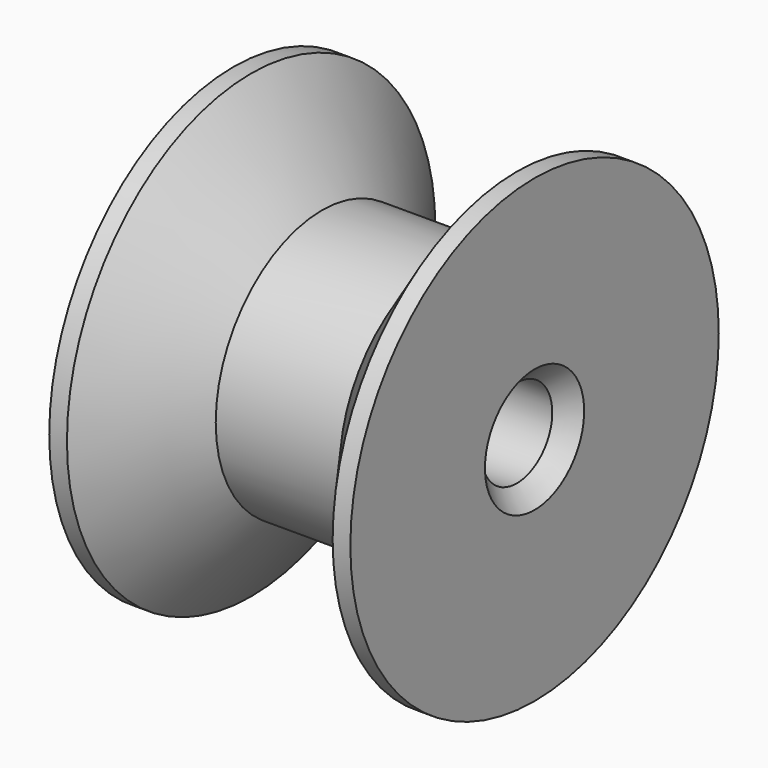
from build123d import *

# Parameters (mm, degrees)
F2_SIZE2 = 10.99999
F2_SIZE  = 7.99999
F3_SIZE  = 2


# Not quite as in the source:
# - a fillet or chamfer is up to 0.001 mm smaller than in the source, because OpenCascade refuses the exact size


with BuildPart() as f1:
    # F0 (on Front) → F1 (revolve)
    with BuildSketch(Plane.XZ):
        Polygon((0, 26), (0, 5), (34, 5), (34, 26), (32, 26), (32, 15), (2, 15), (2, 26), align=None)
    revolve(axis=Axis((17, 0, 0), (1, 0, 0)))

    # F2 (size 8 and 11 in the source; OpenCascade refuses exactly that, so slightly less here)
    f2_edges = [f1.edges().sort_by_distance(p)[0] for p in [
        (2, 0, -15),
        (32, 0, -15),
    ]]
    f2_side = f1.faces().sort_by_distance((17, 0, -15))[0]
    chamfer(f2_edges, length=F2_SIZE, length2=F2_SIZE2, reference=f2_side)

    # F3
    f3_edges = [f1.edges().sort_by_distance(p)[0] for p in [
        (0, 0, -5),
        (34, 0, -5),
    ]]
    chamfer(f3_edges, length=F3_SIZE)


solid = f1.part
